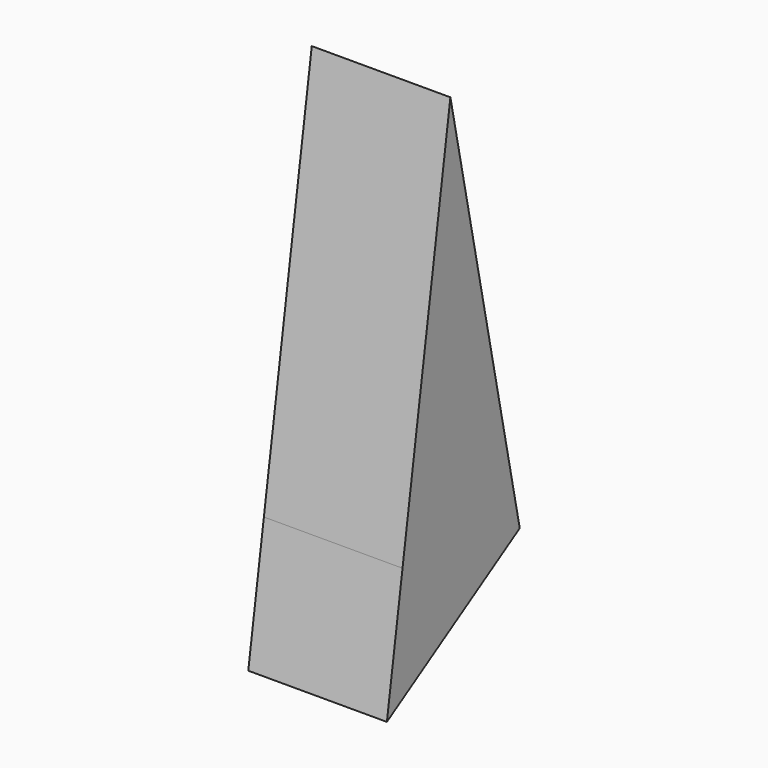
from build123d import *

# Parameters (mm, degrees)
F1_DEPTH = 50.8


# Not quite as in the source:
# - a feature names something its author has since deleted; it is built from what else it names


with BuildPart() as f1:
    # F0 (on Right) → F1 (new body)
    with BuildSketch(Plane.YZ):
        Polygon((99.9464914203, 77.3684754968), (78.0169366286, -65.6313263369), (131.7094862461, -74.5480582118), align=None)
        Polygon((131.7094862461, -74.5480582118), (78.0169366286, -65.6313263369), (70.8601698279, -112.2996807098), align=None)
    extrude(amount=F1_DEPTH)


solid = f1.part
